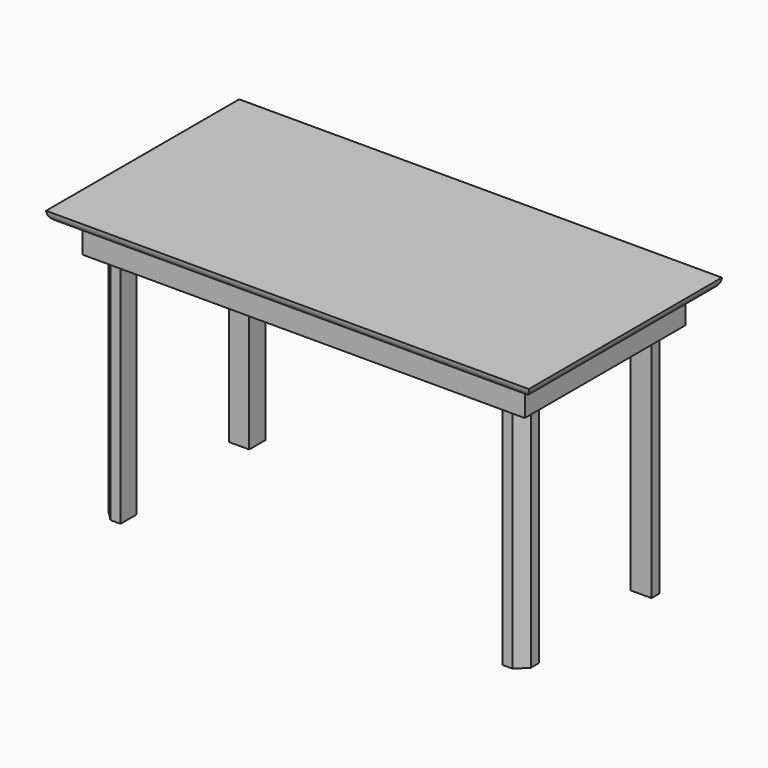
from build123d import *

# Parameters (mm, degrees)
F0_W     = 1219.2
F0_H     = 609.6
F1_DEPTH = 25.4
F2_W     = 1117.6
F2_H     = 508
F2_W_2   = 1066.8
F2_H_2   = 457.2
F3_DEPTH = 76.2
F4_W     = 50.8
F4_H     = 50.8
F4_W_2   = 52.8930136204
F5_DEPTH = 660.4
F6_R     = 25.39999
F7_SIZE  = 25.4


# Not quite as in the source:
# - a fillet or chamfer is up to 0.001 mm smaller than in the source, because OpenCascade refuses the exact size


with BuildPart() as f1:
    # F0 (on Top) → F1 (new body)
    with BuildSketch(Plane.XY):
        Rectangle(F0_W, F0_H)
    extrude(amount=F1_DEPTH)

    # F2 (on face) → F3 (join)
    with BuildSketch(Plane(origin=(0, 0, 0), x_dir=(1, 0, 0), z_dir=(0, 0, -1))):
        Rectangle(F2_W, F2_H)
        Rectangle(F2_W_2, F2_H_2, mode=Mode.SUBTRACT)
    extrude(amount=F3_DEPTH)

    # F4 (on face) → F5 (join)
    with BuildSketch(Plane(origin=(0, 0, 0), x_dir=(1, 0, 0), z_dir=(0, 0, -1))):
        with Locations((-508, 203.2)):
            Rectangle(F4_W, F4_H)
        with Locations((-508, -203.2)):
            Rectangle(F4_W, F4_H)
        with Locations((506.9534931898, -203.2)):
            Rectangle(F4_W_2, F4_H)
        with Locations((508, 203.2)):
            Rectangle(F4_W, F4_H)
    extrude(amount=F5_DEPTH)

    # F6 (radius 25.4 in the source; OpenCascade refuses exactly that, so slightly less here)
    f6_edges = [f1.edges().sort_by_distance(p)[0] for p in [
        (0, 304.8, 0),
        (-609.6, 0, 0),
        (609.6, 0, 0),
        (0, -304.8, 0),
    ]]
    fillet(f6_edges, radius=F6_R)

    # F7
    f7_edges = [f1.edges().sort_by_distance(p)[0] for p in [
        (-533.4, -228.6, -368.3),
        (-533.4, 228.6, -368.3),
        (533.4, 228.6, -368.3),
        (533.4, -228.6, -368.3),
    ]]
    chamfer(f7_edges, length=F7_SIZE)


solid = f1.part
